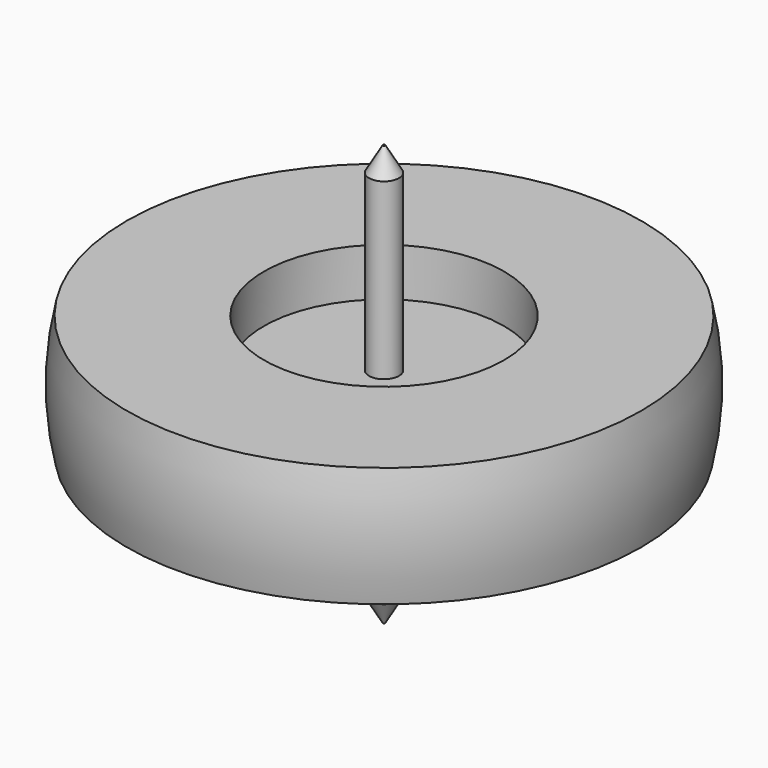
from build123d import *

# Parameters (mm, degrees)
F3_SIZE2 = 2.9329393675
F3_SIZE  = 5.08


# Not quite as in the source:
# - a fillet or chamfer that OpenCascade refuses, or shapes differently, is made with other operations: its cross-section is extruded or revolved along the edge and cut away or added


with BuildPart() as f1:
    # F0 (on Front) → F1 (revolve)
    with BuildSketch(Plane.XZ):
        Polygon((3.175, 44.45), (0, 44.45), (0, 0), (50.8, 0), (50.8, 12.7), (25.478093854, 12.7), (25.4, 12.7), (25.4, 2.54), (3.175, 2.54), align=None)
        Polygon((50.8, 0), (0, 0), (0, -44.45), (3.175, -44.45), (3.175, -2.54), (25.4, -2.54), (25.4, -12.7), (50.8, -12.7), align=None)
    revolve(axis=Axis((0, 0, 0), (0, 0, 1)))

    # F2: chamfer of 5.08 x 2.9329393675 on 1 edges, made by hand

    # F2_s1 → F2_t2 (revolve, cut)
    with BuildSketch(Plane.XZ):
        Polygon((3.175, 39.37), (0.2420606325, 44.45), (3.175, 44.45), align=None)
    revolve(axis=Axis((0, 0, 44.45), (0, 0, 1)), mode=Mode.SUBTRACT)

    # F3
    f3_edges = [f1.edges().sort_by_distance(p)[0] for p in [
        (-3.175, 0, -44.45),
    ]]
    chamfer(f3_edges, length=F3_SIZE, length2=F3_SIZE2)

    # F4 (on Front) → F5 (revolve)
    with BuildSketch(Plane.XZ):
        with BuildLine():
            Line((50.8, -12.7), (54.4176846255, -12.7))
            ThreePointArc((54.4176846255, -12.7), (55.88, 0), (54.4176846255, 12.7))
            Line((54.4176846255, 12.7), (50.8, 12.7))
            Line((50.8, 12.7), (50.8, -12.7))
        make_face()
    revolve(axis=Axis((0, 0, 12.7), (0, 0, 1)))


solid = f1.part
